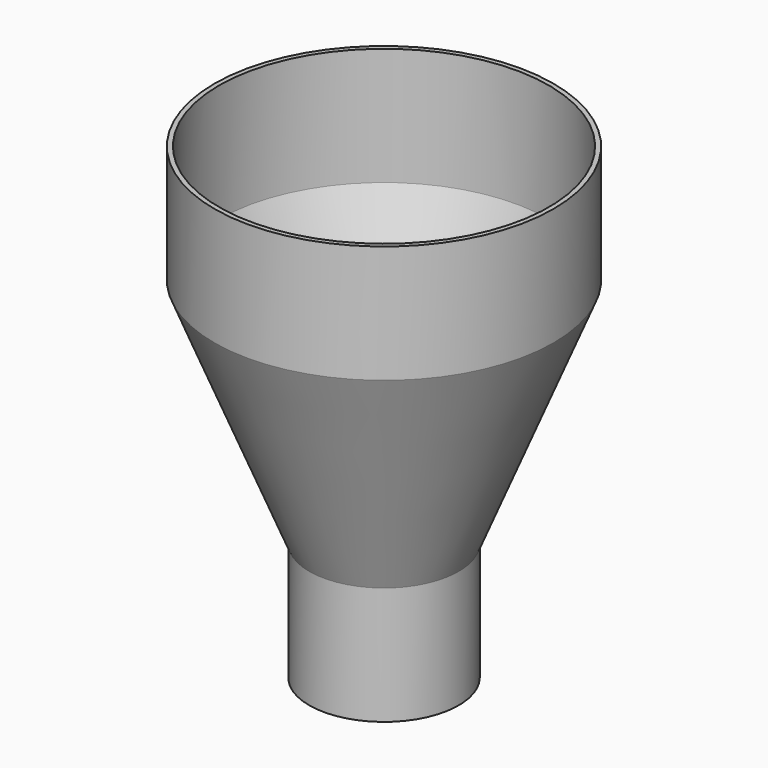
from build123d import *


# Not quite as in the source:
# - ends of sketch curves that miss each other by under 0.0002 mm in the source are joined


with BuildPart() as f1:
    # F0 (on Front) → F1 (revolve)
    with BuildSketch(Plane.XZ):
        Polygon((-15.113, -75.5039413649), (-15.113, -50.1039413649), (-16.1289999974, -50.1038177847), (-16.1289999982, -75.5039413649), align=None)
        Polygon((-15.1129998177, -50.1039412905), (-35.5600012367, -0.0001234082), (-36.5760016743, 7.015e-07), (-16.1290002526, -50.1038178889), align=None)
        Polygon((-36.5760016743, 7.015e-07), (-35.5600012367, -0.0001228868), (-35.56, 25.3998765918), (-36.5759999982, 25.3998765918), align=None)
    revolve(axis=Axis((0, 0, -37.7519706824), (0, 0, -1)))


solid = f1.part
